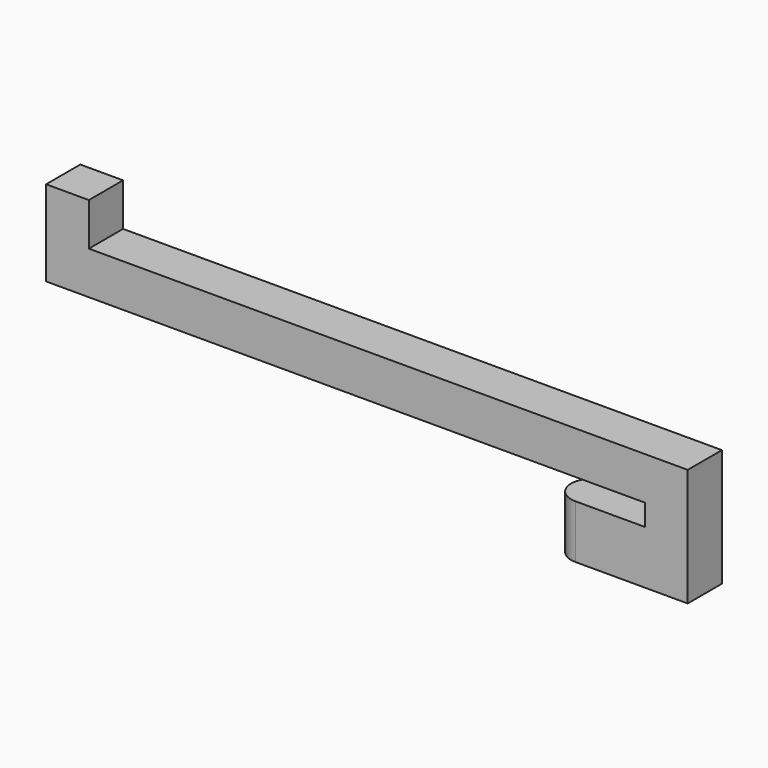
from build123d import *

# Parameters (mm, degrees)
F0_W     = 8
F0_H     = 8
F1_DEPTH = 120
F2_W     = 8
F2_H     = 8
F3_DEPTH = 8
F4_W     = 8
F4_H     = 8
F5_DEPTH = 4
F6_W     = 17
F6_H     = 8
F6_W_2   = 8
F7_DEPTH = 10
F8_R     = 3.99999


# Not quite as in the source:
# - a fillet or chamfer is up to 0.001 mm smaller than in the source, because OpenCascade refuses the exact size


with BuildPart() as f1:
    # F0 (on Right) → F1 (new body)
    with BuildSketch(Plane.YZ):
        Rectangle(F0_W, F0_H)
    extrude(amount=F1_DEPTH)

    # F2 (on face) → F3 (join)
    with BuildSketch(Plane.XY.offset(4)):
        with Locations((4, 0)):
            Rectangle(F2_W, F2_H)
    extrude(amount=F3_DEPTH)

    # F4 (on face) → F5 (join)
    with BuildSketch(Plane(origin=(0, 0, -4), x_dir=(1, 0, 0), z_dir=(0, 0, -1))):
        with Locations((116, 0)):
            Rectangle(F4_W, F4_H)
    extrude(amount=F5_DEPTH)

    # F6 (on face) → F7 (join)
    with BuildSketch(Plane(origin=(0, 0, -8), x_dir=(1, 0, 0), z_dir=(0, 0, -1))):
        with Locations((103.5, 0)):
            Rectangle(F6_W, F6_H)
        with Locations((116, 0)):
            Rectangle(F6_W_2, F6_H)
    extrude(amount=F7_DEPTH)

    # F8 (radius 4 in the source; OpenCascade refuses exactly that, so slightly less here)
    f8_edges = [f1.edges().sort_by_distance(p)[0] for p in [
        (95, -4, -13),
        (95, 4, -13),
    ]]
    fillet(f8_edges, radius=F8_R)


solid = f1.part
